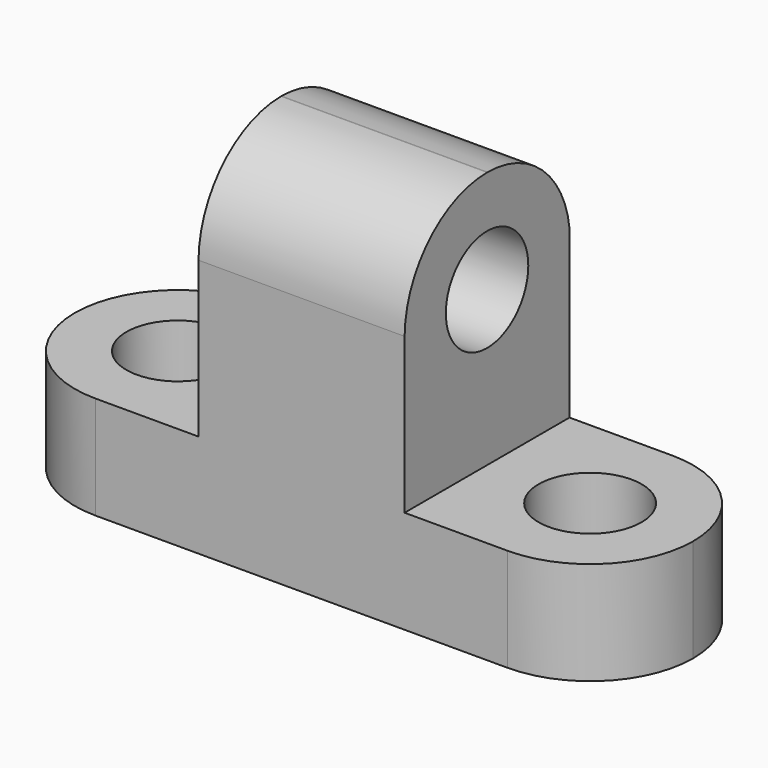
from build123d import *

# Parameters (mm, degrees)
F1_DEPTH = 25.4
F2_R     = 6.35
F3_DEPTH = 25.4
F4_R     = 6.35
F5_DEPTH = 12.7
F7_DEPTH = 12.7


# Not quite as in the source:
# - ends of sketch curves that miss each other by under 0.0002 mm in the source are joined


with BuildPart() as f1:
    # F0 (on Front) → F1 (new body)
    with BuildSketch(Plane.XZ):
        Polygon((0, 12.7), (0, 0), (76.2, 0), (76.2, 12.7), (50.8, 12.7), (50.8, 44.45), (25.4, 44.45), (25.4, 12.7), align=None)
    extrude(amount=F1_DEPTH)

    # F2 (on face) → F3 (cut)
    with BuildSketch(Plane.YZ.offset(50.8)):
        with Locations((-12.7, 31.75)):
            Circle(F2_R)
        with BuildLine():
            ThreePointArc((-12.6538738539, 44.4500834572), (-4.2011824857, 41.2444061447), (0, 33.2397559887))
            Line((0, 33.2397559887), (0, 44.45))
            Line((0, 44.45), (-12.6538738539, 44.4500834572))
        make_face()
        with BuildLine():
            ThreePointArc((-25.4, 31.8358913064), (-21.6202217079, 40.7633957722), (-12.6538738539, 44.4500834572))
            Line((-12.6538738539, 44.4500834572), (-25.4, 44.45))
            Line((-25.4, 44.45), (-25.4, 31.8358913064))
        make_face()
    extrude(amount=-F3_DEPTH, mode=Mode.SUBTRACT)

    # F4 (on face) → F5 (cut)
    with BuildSketch(Plane.XY.offset(12.7)):
        with Locations((12.7003350629, -12.6999999956)):
            Circle(F4_R)
        with BuildLine():
            ThreePointArc((0, -12.7), (3.7197438789, -3.7197438789), (12.7, 0))
            Line((12.7, 0), (0, 0))
            Line((0, 0), (0, -12.7))
        make_face()
        with Locations((63.5, -12.7)):
            Circle(F4_R)
        with BuildLine():
            Line((0, -25.4), (12.7, -25.4))
            ThreePointArc((12.7, -25.4), (3.7197438789, -21.6802561211), (0, -12.7))
            Line((0, -12.7), (0, -25.4))
        make_face()
    extrude(amount=-F5_DEPTH, mode=Mode.SUBTRACT)

    # F6 (on face) → F7 (cut)
    with BuildSketch(Plane.XY.offset(12.7)):
        with BuildLine():
            ThreePointArc((76.2000025586, -12.7), (72.4802576974, -21.6802565734), (63.5, -25.3999987207))
            Line((63.5, -25.3999987207), (76.2, -25.4))
            Line((76.2, -25.4), (76.2000025586, -12.7))
        make_face()
        with BuildLine():
            ThreePointArc((63.5, -1.2793e-06), (72.4802576975, -3.7197434266), (76.2000025586, -12.7))
            Line((76.2000025586, -12.7), (76.2, 0))
            Line((76.2, 0), (63.5, -1.2793e-06))
        make_face()
    extrude(amount=-F7_DEPTH, mode=Mode.SUBTRACT)


solid = f1.part
